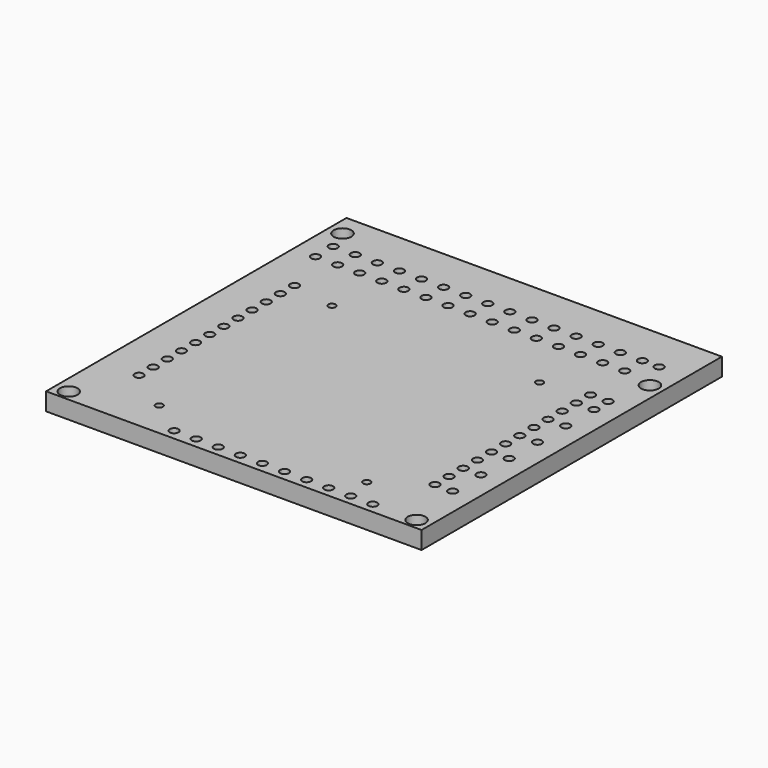
from build123d import *

# Parameters (mm, degrees)
F0_W     = 170
F0_H     = 170
F0_R     = 2
F0_R_2   = 1.65
F1_DEPTH = 8
F2_R     = 4
F2_R_2   = 2
F3_DEPTH = 6


with BuildPart() as f1:
    # F0 (on Top) → F1 (new body)
    with BuildSketch(Plane.XY):
        with Locations((85, -85)):
            Rectangle(F0_W, F0_H)
        with Locations((6.35, -165.1)):
            Circle(F0_R, mode=Mode.SUBTRACT)
        with Locations((18, -139.89)):
            Circle(F0_R, mode=Mode.SUBTRACT)
        with Locations((18, -131.89)):
            Circle(F0_R, mode=Mode.SUBTRACT)
        with Locations((54.2, -165.3)):
            Circle(F0_R, mode=Mode.SUBTRACT)
        with Locations((64.2, -165.3)):
            Circle(F0_R, mode=Mode.SUBTRACT)
        with Locations((74.2, -165.3)):
            Circle(F0_R, mode=Mode.SUBTRACT)
        with Locations((38.01, -153.49)):
            Circle(F0_R_2, mode=Mode.SUBTRACT)
        with Locations((18, -123.89)):
            Circle(F0_R, mode=Mode.SUBTRACT)
        with Locations((18, -115.89)):
            Circle(F0_R, mode=Mode.SUBTRACT)
        with Locations((18, -107.89)):
            Circle(F0_R, mode=Mode.SUBTRACT)
        with Locations((18, -99.89)):
            Circle(F0_R, mode=Mode.SUBTRACT)
        with Locations((18, -91.89)):
            Circle(F0_R, mode=Mode.SUBTRACT)
        with Locations((18, -83.89)):
            Circle(F0_R, mode=Mode.SUBTRACT)
        with Locations((84.2, -165.3)):
            Circle(F0_R, mode=Mode.SUBTRACT)
        with Locations((94.2, -165.3)):
            Circle(F0_R, mode=Mode.SUBTRACT)
        with Locations((104.2, -165.3)):
            Circle(F0_R, mode=Mode.SUBTRACT)
        with Locations((114.2, -165.3)):
            Circle(F0_R, mode=Mode.SUBTRACT)
        with Locations((124.2, -165.3)):
            Circle(F0_R, mode=Mode.SUBTRACT)
        with Locations((134.2, -165.3)):
            Circle(F0_R, mode=Mode.SUBTRACT)
        with Locations((131.99, -153.49)):
            Circle(F0_R_2, mode=Mode.SUBTRACT)
        with Locations((144.2, -165.3)):
            Circle(F0_R, mode=Mode.SUBTRACT)
        with Locations((163.83, -165.1)):
            Circle(F0_R, mode=Mode.SUBTRACT)
        with Locations((152, -139.89)):
            Circle(F0_R, mode=Mode.SUBTRACT)
        with Locations((152, -131.89)):
            Circle(F0_R, mode=Mode.SUBTRACT)
        with Locations((160, -139.89)):
            Circle(F0_R, mode=Mode.SUBTRACT)
        with Locations((152, -123.89)):
            Circle(F0_R, mode=Mode.SUBTRACT)
        with Locations((160, -123.89)):
            Circle(F0_R, mode=Mode.SUBTRACT)
        with Locations((152, -115.89)):
            Circle(F0_R, mode=Mode.SUBTRACT)
        with Locations((152, -107.89)):
            Circle(F0_R, mode=Mode.SUBTRACT)
        with Locations((160, -107.89)):
            Circle(F0_R, mode=Mode.SUBTRACT)
        with Locations((152, -99.89)):
            Circle(F0_R, mode=Mode.SUBTRACT)
        with Locations((152, -91.89)):
            Circle(F0_R, mode=Mode.SUBTRACT)
        with Locations((152, -83.89)):
            Circle(F0_R, mode=Mode.SUBTRACT)
        with Locations((160, -91.89)):
            Circle(F0_R, mode=Mode.SUBTRACT)
        with Locations((18, -75.89)):
            Circle(F0_R, mode=Mode.SUBTRACT)
        with Locations((18, -67.89)):
            Circle(F0_R, mode=Mode.SUBTRACT)
        with Locations((18, -59.89)):
            Circle(F0_R, mode=Mode.SUBTRACT)
        with Locations((18, -51.89)):
            Circle(F0_R, mode=Mode.SUBTRACT)
        with Locations((38.01, -55.7)):
            Circle(F0_R_2, mode=Mode.SUBTRACT)
        with Locations((10, -30)):
            Circle(F0_R, mode=Mode.SUBTRACT)
        with Locations((20, -30)):
            Circle(F0_R, mode=Mode.SUBTRACT)
        with Locations((10, -20)):
            Circle(F0_R, mode=Mode.SUBTRACT)
        with Locations((20, -20)):
            Circle(F0_R, mode=Mode.SUBTRACT)
        with Locations((6.35, -10.16)):
            Circle(F0_R, mode=Mode.SUBTRACT)
        with Locations((30, -30)):
            Circle(F0_R, mode=Mode.SUBTRACT)
        with Locations((30, -20)):
            Circle(F0_R, mode=Mode.SUBTRACT)
        with Locations((40, -30)):
            Circle(F0_R, mode=Mode.SUBTRACT)
        with Locations((50, -30)):
            Circle(F0_R, mode=Mode.SUBTRACT)
        with Locations((40, -20)):
            Circle(F0_R, mode=Mode.SUBTRACT)
        with Locations((50, -20)):
            Circle(F0_R, mode=Mode.SUBTRACT)
        with Locations((60, -30)):
            Circle(F0_R, mode=Mode.SUBTRACT)
        with Locations((60, -20)):
            Circle(F0_R, mode=Mode.SUBTRACT)
        with Locations((70, -30)):
            Circle(F0_R, mode=Mode.SUBTRACT)
        with Locations((80, -30)):
            Circle(F0_R, mode=Mode.SUBTRACT)
        with Locations((70, -20)):
            Circle(F0_R, mode=Mode.SUBTRACT)
        with Locations((80, -20)):
            Circle(F0_R, mode=Mode.SUBTRACT)
        with Locations((131.99, -55.7)):
            Circle(F0_R_2, mode=Mode.SUBTRACT)
        with Locations((152, -75.89)):
            Circle(F0_R, mode=Mode.SUBTRACT)
        with Locations((160, -75.89)):
            Circle(F0_R, mode=Mode.SUBTRACT)
        with Locations((152, -67.89)):
            Circle(F0_R, mode=Mode.SUBTRACT)
        with Locations((152, -59.89)):
            Circle(F0_R, mode=Mode.SUBTRACT)
        with Locations((160, -59.89)):
            Circle(F0_R, mode=Mode.SUBTRACT)
        with Locations((152, -51.89)):
            Circle(F0_R, mode=Mode.SUBTRACT)
        with Locations((160, -51.89)):
            Circle(F0_R, mode=Mode.SUBTRACT)
        with Locations((163.83, -33.02)):
            Circle(F0_R, mode=Mode.SUBTRACT)
        with Locations((90, -30)):
            Circle(F0_R, mode=Mode.SUBTRACT)
        with Locations((90, -20)):
            Circle(F0_R, mode=Mode.SUBTRACT)
        with Locations((100, -30)):
            Circle(F0_R, mode=Mode.SUBTRACT)
        with Locations((110, -30)):
            Circle(F0_R, mode=Mode.SUBTRACT)
        with Locations((100, -20)):
            Circle(F0_R, mode=Mode.SUBTRACT)
        with Locations((110, -20)):
            Circle(F0_R, mode=Mode.SUBTRACT)
        with Locations((120, -30)):
            Circle(F0_R, mode=Mode.SUBTRACT)
        with Locations((120, -20)):
            Circle(F0_R, mode=Mode.SUBTRACT)
        with Locations((130, -30)):
            Circle(F0_R, mode=Mode.SUBTRACT)
        with Locations((130, -20)):
            Circle(F0_R, mode=Mode.SUBTRACT)
        with Locations((140, -30)):
            Circle(F0_R, mode=Mode.SUBTRACT)
        with Locations((150, -30)):
            Circle(F0_R, mode=Mode.SUBTRACT)
        with Locations((140, -20)):
            Circle(F0_R, mode=Mode.SUBTRACT)
        with Locations((150, -20)):
            Circle(F0_R, mode=Mode.SUBTRACT)
        with Locations((157.560000028, -20)):
            Circle(F0_R, mode=Mode.SUBTRACT)
    extrude(amount=F1_DEPTH)

    # F2 (on face) → F3 (cut)
    with BuildSketch(Plane.XY.offset(8)):
        with Locations((163.83, -33.02)):
            Circle(F2_R)
        with Locations((163.83, -33.02)):
            Circle(F2_R_2, mode=Mode.SUBTRACT)
        with Locations((163.83, -165.1)):
            Circle(F2_R)
        with Locations((163.83, -165.1)):
            Circle(F2_R_2, mode=Mode.SUBTRACT)
        with Locations((6.35, -165.1)):
            Circle(F2_R)
        with Locations((6.35, -165.1)):
            Circle(F2_R_2, mode=Mode.SUBTRACT)
        with Locations((6.35, -10.16)):
            Circle(F2_R)
        with Locations((6.35, -10.16)):
            Circle(F2_R_2, mode=Mode.SUBTRACT)
    extrude(amount=-F3_DEPTH, mode=Mode.SUBTRACT)


solid = f1.part
